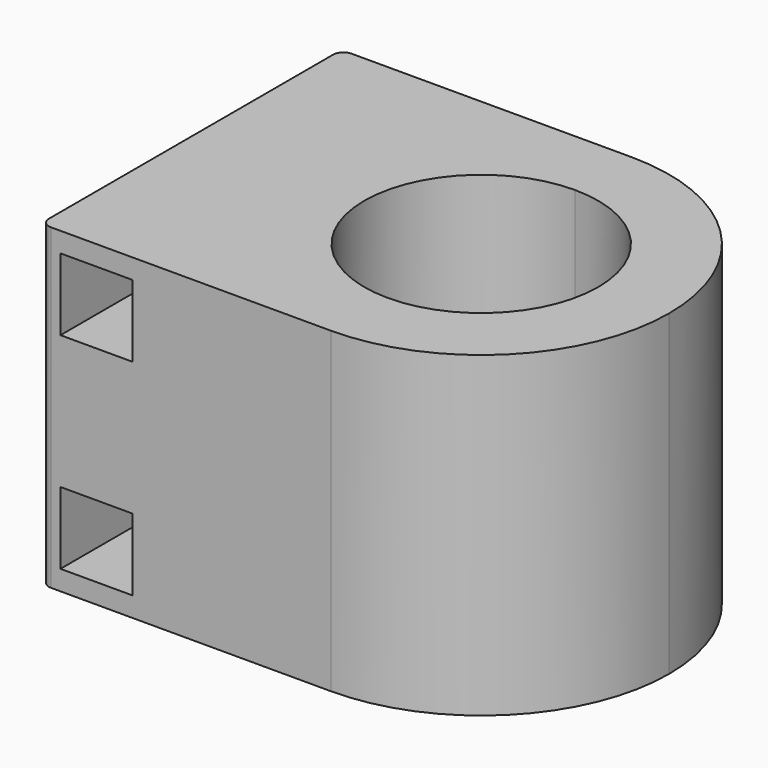
from build123d import *

# Parameters (mm, degrees)
F1_DEPTH = 30.4
F2_DEPTH = 2
F3_W     = 6.9
F3_H     = 6.9
F4_DEPTH = 50
F5_R     = 1


# Not quite as in the source:
# - a feature of the source that left no trace in its solid (it failed there, or was rolled back) is left out
# - a feature names something its author has since deleted; it is built from what else it names


with BuildPart() as f1:
    # F0 (on Top) → F1 (new body)
    with BuildSketch(Plane.XY):
        with BuildLine():
            ThreePointArc((0, -18), (-18, 0), (0, 18))
            Line((0, 18), (-27.8, 18))
            Line((-27.8, 18), (-27.8, -18))
            Line((-27.8, -18), (0, -18))
        make_face()
        with BuildLine():
            ThreePointArc((0, -11.2), (-11.2, 0), (0, 11.2))
            Line((0, 11.2), (0, 18))
            ThreePointArc((0, 18), (-18, 0), (0, -18))
            Line((0, -18), (0, -11.2))
        make_face()
        with BuildLine():
            ThreePointArc((0, 11.2), (7.9195959493, 7.9195959493), (11.2, 0))
            ThreePointArc((11.2, 0), (7.9195959493, -7.9195959493), (0, -11.2))
            Line((0, -11.2), (0, -18))
            ThreePointArc((0, -18), (12.7279220614, -12.7279220614), (18, 0))
            ThreePointArc((18, 0), (12.7279220614, 12.7279220614), (0, 18))
            Line((0, 18), (0, 11.2))
        make_face()
    extrude(amount=F1_DEPTH)

    # F0 (on Top) → F2 (join)
    with BuildSketch(Plane.XY):
        with BuildLine():
            ThreePointArc((0, -11.2), (7.9195959493, -7.9195959493), (11.2, 0))
            ThreePointArc((11.2, 0), (7.9195959493, 7.9195959493), (0, 11.2))
            Line((0, 11.2), (0, 5))
            ThreePointArc((0, 5), (3.5355339059, 3.5355339059), (5, 0))
            ThreePointArc((5, 0), (3.5355339059, -3.5355339059), (0, -5))
            Line((0, -5), (0, -11.2))
        make_face()
        with BuildLine():
            Line((0, 5), (0, 11.2))
            ThreePointArc((0, 11.2), (-11.2, 0), (0, -11.2))
            Line((0, -11.2), (0, -5))
            ThreePointArc((0, -5), (-5, 0), (0, 5))
        make_face()
    extrude(amount=F2_DEPTH)

    # F3 (on face) → F4 (cut)
    with BuildSketch(Plane.XZ.offset(18)):
        with Locations((-22.45, 25.05)):
            Rectangle(F3_W, F3_H)
        with Locations((-22.45, 5.35)):
            Rectangle(F3_W, F3_H)
    extrude(amount=-F4_DEPTH, mode=Mode.SUBTRACT)

    # F5
    f5_edges = [f1.edges().sort_by_distance(p)[0] for p in [
        (-27.8, 18, 15.2),
        (-27.8, -18, 15.2),
    ]]
    fillet(f5_edges, radius=F5_R)


solid = f1.part
